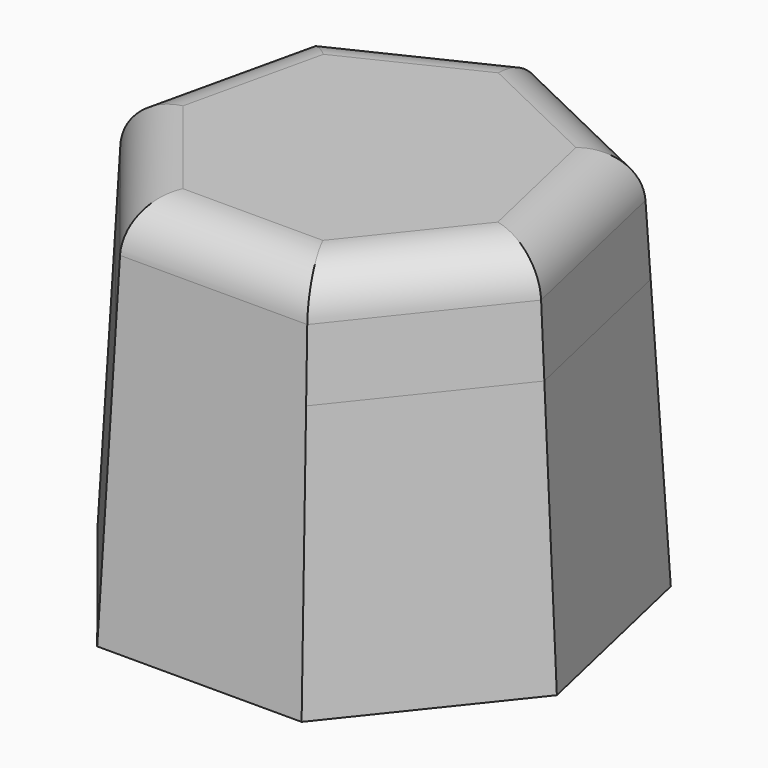
from build123d import *

# Parameters (mm, degrees)
F1_DEPTH      = 25
F1_TAPER      = 3
F1_DEPTH_BACK = 58.2
F1_TAPER_BACK = -3
F2_R          = 10.5652829809
F3_T          = -2.5


with BuildPart() as f1:
    # F0 (on Top) → F1 (new body, two sides)
    with BuildSketch(Plane.XY) as f1_sk:
        Polygon((-20.5419126951, -42.6557212379), (20.5419126951, -42.6557212379), (46.1572588473, -10.5350931276), (37.0152476509, 29.5186749845), (0, 47.3442787621), (-37.0152476509, 29.5186749845), (-46.1572588473, -10.5350931276), align=None)
    extrude(amount=F1_DEPTH, taper=F1_TAPER)
    extrude(f1_sk.sketch, amount=-F1_DEPTH_BACK, taper=F1_TAPER_BACK)

    # F2
    f2_edges = [f1.edges().sort_by_distance(p)[0] for p in [
        (-32.325234, -25.778514, 25),
        (0, -41.345527, 25),
        (32.325234, -25.778514, 25),
        (40.308908, 9.200245, 25),
        (17.939152, 37.251032, 25),
        (-17.939152, 37.251032, 25),
        (-40.308908, 9.200245, 25),
    ]]
    fillet(f2_edges, radius=F2_R)

    # F3
    f3_openings = [f1.faces().sort_by_distance(p)[0] for p in [
        (0, 0, -58.2),
    ]]
    offset(amount=F3_T, openings=f3_openings)


solid = f1.part
